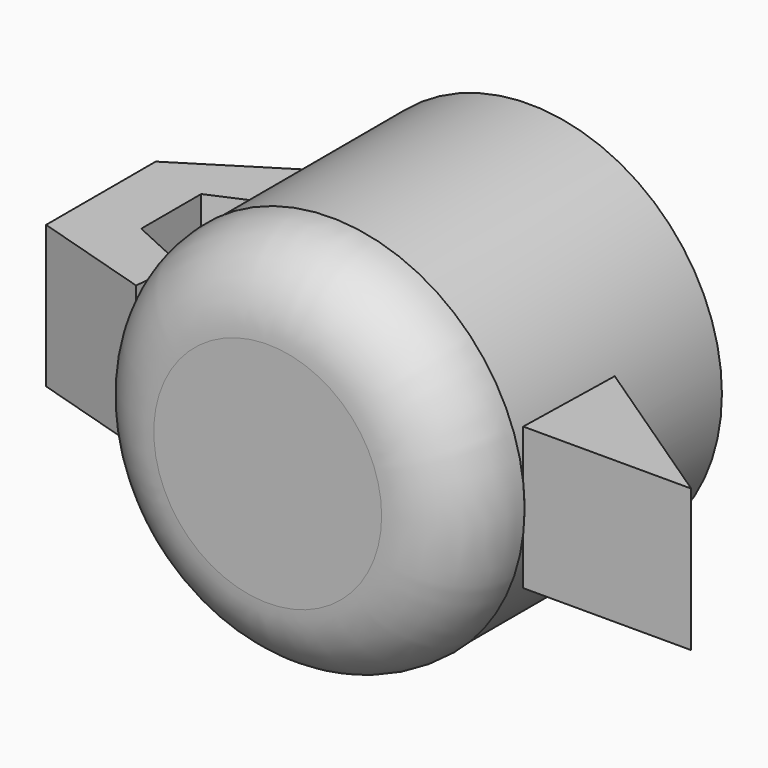
from build123d import *

# Parameters (mm, degrees)
F0_R     = 34.3734140818
F1_DEPTH = 44.2854
F2_R     = 34.5672113186
F3_DEPTH = 14.14017
F6_DEPTH = 12.7
F8_DEPTH = 12.7


# Not quite as in the source:
# - a fillet or chamfer that OpenCascade refuses, or shapes differently, is made with other operations: its cross-section is extruded or revolved along the edge and cut away or added


with BuildPart() as f1:
    # F0 (on Front) → F1 (new body)
    with BuildSketch(Plane.XZ):
        Circle(F0_R)
    extrude(amount=F1_DEPTH)

    # F2 (on face) → F3 (join)
    with BuildSketch(Plane.XZ.offset(44.2854)):
        Circle(F2_R)
    extrude(amount=F3_DEPTH)

    # F4: fillet of radius 14.2211905527 on 1 edges, made by hand

    # F4_s1 → F4_t2 (revolve, cut)
    with BuildSketch(Plane.XY):
        with BuildLine():
            ThreePointArc((34.5672113186, -44.2043794473), (30.4019210422, -54.2602797237), (20.3460207659, -58.42557))
            Line((20.3460207659, -58.42557), (34.5672113186, -58.42557))
            Line((34.5672113186, -58.42557), (34.5672113186, -44.2043794473))
        make_face()
    revolve(axis=Axis((0, -58.42557, 0), (0, -1, 0)), mode=Mode.SUBTRACT)

    # F5 (on Top) → F6 (join, symmetric)
    with BuildSketch(Plane.XY):
        Polygon((34.6197038889, -24.2337957025), (34.1581068933, -44.0824255347), (64.1618520021, -44.0824255347), align=None)
    extrude(amount=F6_DEPTH, both=True)

    # F7 (on Top) → F8 (join, symmetric)
    with BuildSketch(Plane.XY):
        Polygon((-55.8531209826, -38.0816757679), (-34.6197001636, -44.544018805), (-33.6965061724, -35.7736945152), (-44.7748154402, -30.6961387396), (-44.7748154402, -17.3098519444), (-34.158103168, -12.6938922331), (-34.158103168, 0), (-55.8531209826, -13.6170834303), align=None)
    extrude(amount=F8_DEPTH, both=True)


solid = f1.part
